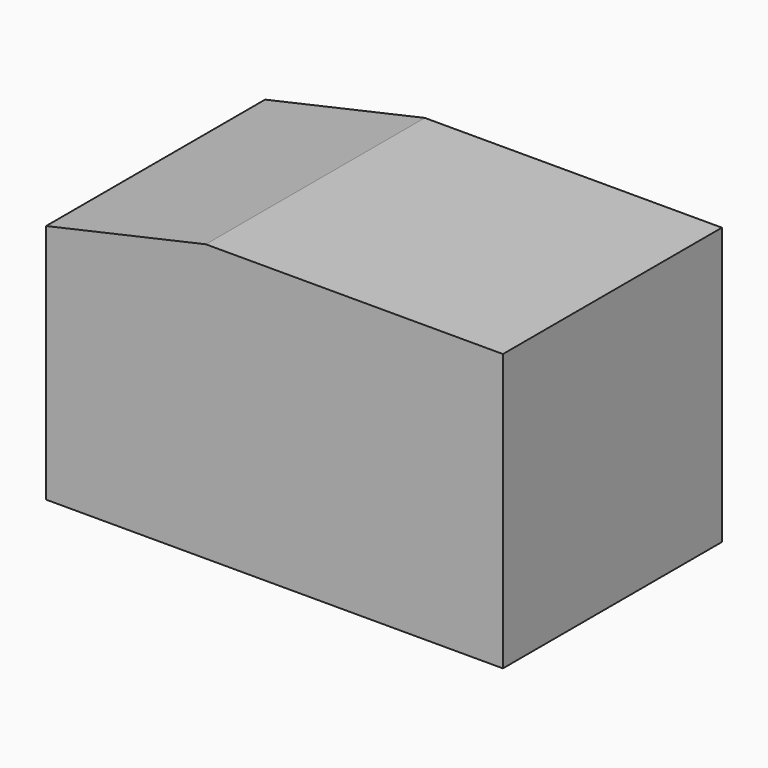
from build123d import *

# Parameters (mm, degrees)
F0_W     = 142.4299553037
F0_H     = 86.2796865404
F1_DEPTH = 85.344
F3_DEPTH = 101.6


# Not quite as in the source:
# - a feature names something its author has since deleted; it is built from what else it names


with BuildPart() as f1:
    # F0 (on Front) → F1 (new body)
    with BuildSketch(Plane.XZ):
        with Locations((4.9032084644, -0.4562679678)):
            Rectangle(F0_W, F0_H)
    extrude(amount=F1_DEPTH)

    # F2 (on face) → F3 (cut)
    with BuildSketch(Plane(origin=(0, 0, 0), x_dir=(-1, 0, 0), z_dir=(0, 1, 0))):
        Polygon((16.5192298591, 42.6835753024), (66.3117691875, 31.5074361861), (66.3117691875, 42.6835753024), align=None)
    extrude(amount=-F3_DEPTH, mode=Mode.SUBTRACT)


solid = f1.part
